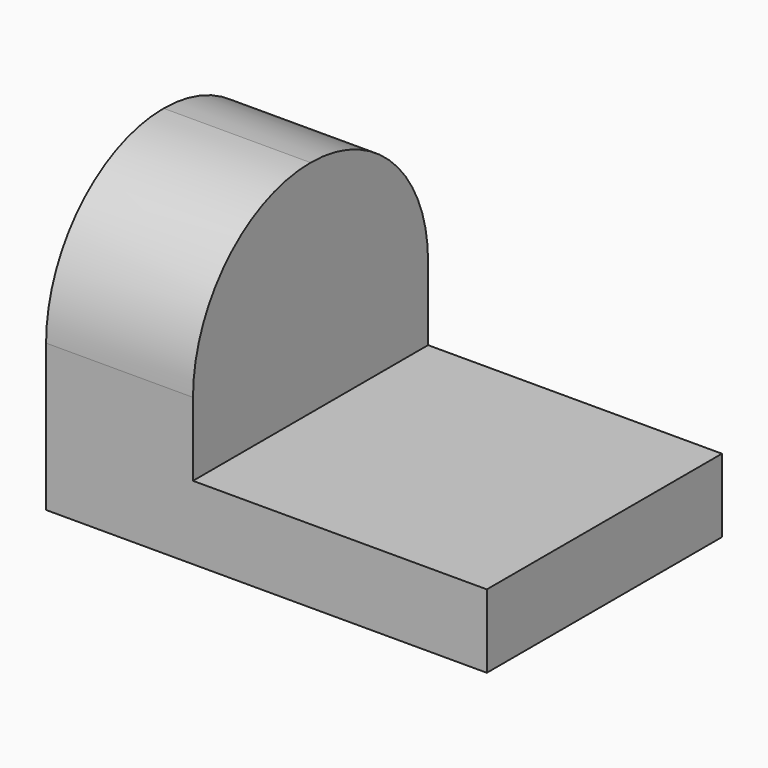
from build123d import *

# Parameters (mm, degrees)
F1_DEPTH = 25.4
F2_R     = 12.69999


# Not quite as in the source:
# - a fillet or chamfer is up to 0.001 mm smaller than in the source, because OpenCascade refuses the exact size


with BuildPart() as f1:
    # F0 (on Front) → F1 (new body)
    with BuildSketch(Plane.XZ):
        Polygon((0, 25.4), (0, 0), (38.1, 0), (38.1, 6.35), (12.7, 6.35), (12.7, 25.4), align=None)
    extrude(amount=-F1_DEPTH)

    # F2 (radius 12.7 in the source; OpenCascade refuses exactly that, so slightly less here)
    f2_edges = [f1.edges().sort_by_distance(p)[0] for p in [
        (6.35, 0, 25.4),
        (6.35, 25.4, 25.4),
    ]]
    fillet(f2_edges, radius=F2_R)


solid = f1.part
